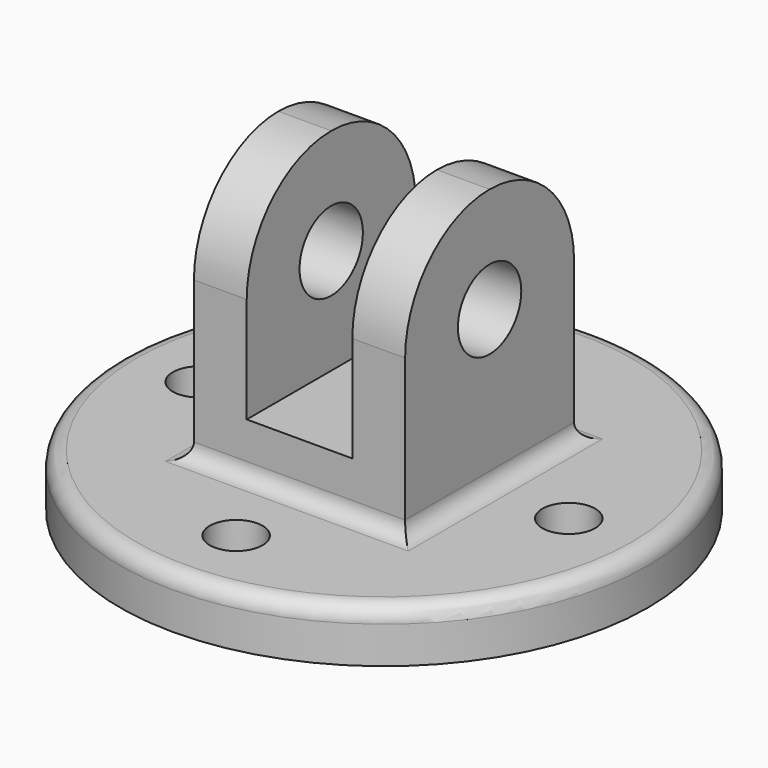
from build123d import *

# Parameters (mm, degrees)
F0_R          = 63.5
F0_R_2        = 6.35
F1_DEPTH      = 12.7
F3_DEPTH      = 25.4
F3_DEPTH_BACK = 25.4
F4_R          = 9.525
F5_DEPTH      = 88.901
F6_DEPTH      = 88.901
F7_R          = 3.81
F8_R          = 3.81


# Not quite as in the source:
# - a feature names something its author has since deleted; it is built from what else it names


with BuildPart() as f1:
    # F0 (on Top) → F1 (new body)
    with BuildSketch(Plane.XY):
        Circle(F0_R)
        with Locations((0, -44.45)):
            Circle(F0_R_2, mode=Mode.SUBTRACT)
        with Locations((-44.45, 0)):
            Circle(F0_R_2, mode=Mode.SUBTRACT)
        with Locations((44.45, 0)):
            Circle(F0_R_2, mode=Mode.SUBTRACT)
        with Locations((0, 44.45)):
            Circle(F0_R_2, mode=Mode.SUBTRACT)
    extrude(amount=F1_DEPTH)

    # F2 (on Front) → F3 (join, two sides)
    with BuildSketch(Plane.XZ) as f3_sk:
        Polygon((-25.4, 0), (0, 0), (25.4, 0), (25.4, 76.2), (12.7, 76.2), (12.7, 25.4), (0, 25.4), (-12.7, 25.4), (-12.7, 76.2), (-25.4, 76.2), align=None)
    extrude(amount=F3_DEPTH)
    extrude(f3_sk.sketch, amount=-F3_DEPTH_BACK)

    # F4 (on face) → F5 (cut, through all)
    with BuildSketch(Plane.YZ.offset(25.4)):
        with Locations((0, 50.8)):
            Circle(F4_R)
    extrude(amount=-F5_DEPTH, mode=Mode.SUBTRACT)

    # F4 (on face) → F6 (cut, through all)
    with BuildSketch(Plane.YZ.offset(25.4)):
        with BuildLine():
            Line((-25.4, 76.2), (-25.4, 50.8))
            ThreePointArc((-25.4, 50.8), (-17.9605122421, 68.7605122421), (0, 76.2))
            Line((0, 76.2), (-25.4, 76.2))
        make_face()
        with BuildLine():
            Line((25.4, 76.2), (0, 76.2))
            ThreePointArc((0, 76.2), (17.9605122421, 68.7605122421), (25.4, 50.8))
            Line((25.4, 50.8), (25.4, 76.2))
        make_face()
    extrude(amount=-F6_DEPTH, mode=Mode.SUBTRACT)

    # F7
    f7_edges = [f1.edges().sort_by_distance(p)[0] for p in [
        (-63.5, 0, 12.7),
    ]]
    fillet(f7_edges, radius=F7_R)

    # F8
    f8_edges = [f1.edges().sort_by_distance(p)[0] for p in [
        (0, -25.4, 12.7),
        (25.4, 0, 12.7),
        (0, 25.4, 12.7),
        (-25.4, 0, 12.7),
    ]]
    fillet(f8_edges, radius=F8_R)


solid = f1.part
